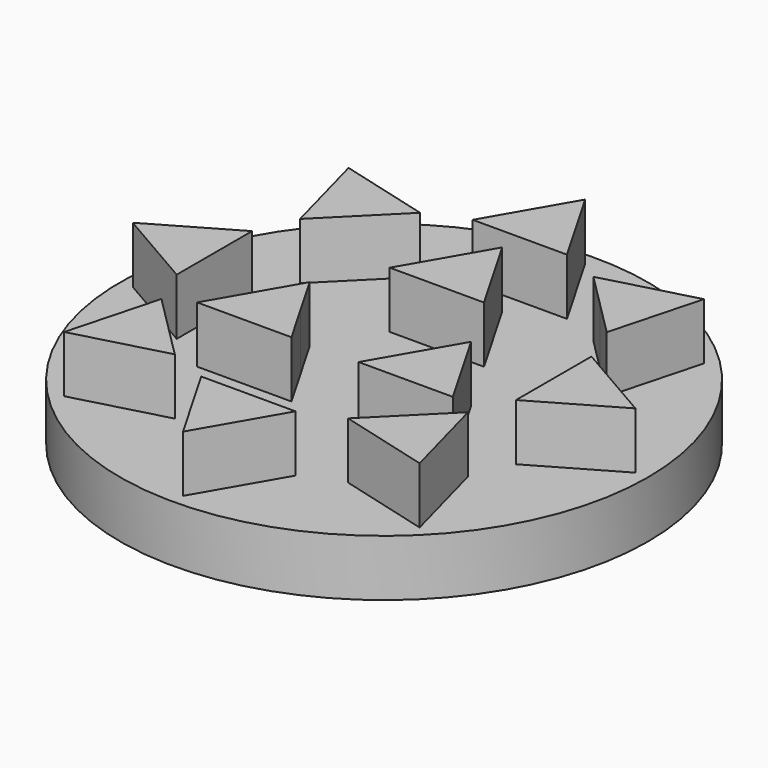
from build123d import *

# Parameters (mm, degrees)
F0_R     = 14
F1_DEPTH = 3
F3_DEPTH = 3
F4_SCALE = 0.7143


# Not quite as in the source:
# - a feature names something its author has since deleted; it is built from what else it names


with BuildPart() as f1:
    # F0 (on Top) → F1 (new body)
    with BuildSketch(Plane.XY):
        Circle(F0_R)
    extrude(amount=F1_DEPTH)

    # F2 (on face) → F3 (join)
    with BuildSketch(Plane.XY.offset(3)):
        Polygon((0, 3.5), (2.5, 3.5), (0, 7.8301270189), (-2.5, 3.5), align=None)
        Polygon((-1.7810889132, -3.9150635095), (-3.0310888244, -1.7500001539), (-4.2810889132, 0.4150635095), (-6.7810889132, -3.9150635095), align=None)
        Polygon((4.2810889132, 0.4150635095), (3.0310888244, -1.7500001539), (1.7810889132, -3.9150635095), (6.7810889132, -3.9150635095), align=None)
        Polygon((-8.1317279836, 4.5961940777), (-6.3639610341, 6.3639610272), (-4.5961940777, 8.1317279836), (-9.4258232092, 9.4258232092), align=None)
        Polygon((0, 9), (2.5, 9), (0, 13.3301270189), (-2.5, 9), align=None)
        Polygon((4.5961940777, 8.1317279836), (6.3639610512, 6.3639610102), (8.1317279836, 4.5961940777), (9.4258232092, 9.4258232092), align=None)
        Polygon((9, 2.5), (9, 0), (9, -2.5), (13.3301270189, 0), align=None)
        Polygon((8.1317279836, -4.5961940777), (6.3639610307, -6.3639610307), (4.5961940777, -8.1317279836), (9.4258232092, -9.4258232092), align=None)
        Polygon((2.5, -9), (0, -9), (-2.5, -9), (0, -13.3301270189), align=None)
        Polygon((-4.5961940777, -8.1317279836), (-6.3639610486, -6.3639610128), (-8.1317279836, -4.5961940777), (-9.4258232092, -9.4258232092), align=None)
        Polygon((-9, -2.5), (-9, 0), (-9, 2.5), (-13.3301270189, 0), align=None)
    extrude(amount=F3_DEPTH)


with BuildPart() as f1_1:
    # F4: moved
    add(f1.part.scale(F4_SCALE))


solid = f1_1.part
